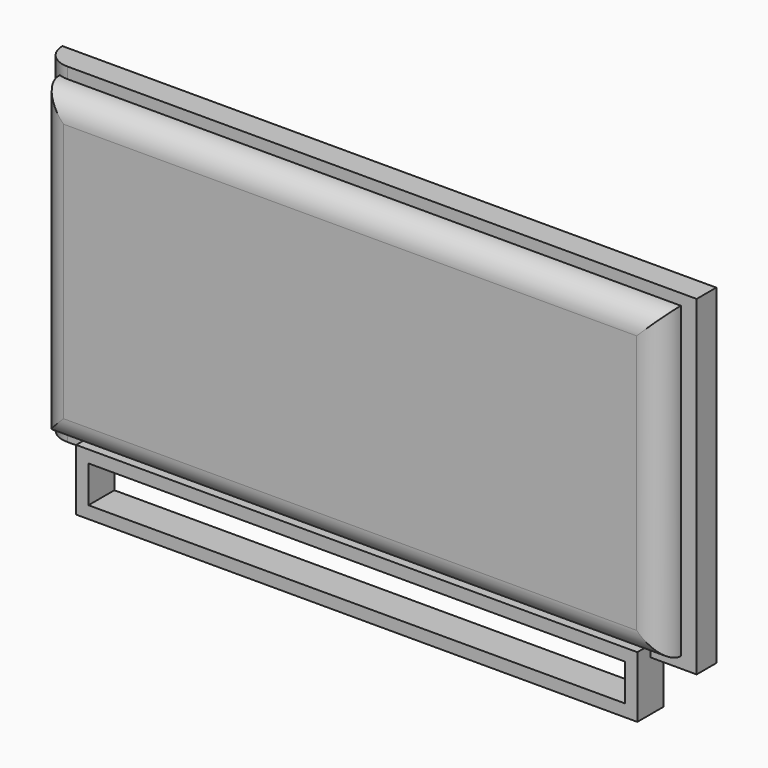
from build123d import *

# Parameters (mm, degrees)
F0_W          = 128.7825703621
F0_H          = 63.8163611293
F1_DEPTH      = 5.08
F0_W_2        = 135.2983415127
F0_H_2        = 68.4157386422
F2_DEPTH      = 5.08
F3_W          = 116.1342710257
F3_H          = 6.7074256949
F4_DEPTH      = 12.7
F5_T          = -2.54
F6_T1_DEPTH   = 89.2163611293
F6_T3_DEPTH   = 154.1825703621
F6_2_T1_DEPTH = 93.8157386422
F7_DEPTH      = 2.54


# Not quite as in the source:
# - a fillet or chamfer that OpenCascade refuses, or shapes differently, is made with other operations: its cross-section is extruded or revolved along the edge and cut away or added


with BuildPart() as f1:
    # F0 (on Front) → F1 (new body)
    with BuildSketch(Plane.XZ):
        Rectangle(F0_W, F0_H)
    extrude(amount=F1_DEPTH)

    # F6: fillet of radius 5.08 on 4 edges, made by hand

    # F6_s2 → F6_t1 (cut)
    with BuildSketch(Plane.XY.offset(-44.6081805646)):
        with BuildLine():
            ThreePointArc((64.391285181, 0), (62.9033876295, -3.5921024484), (59.311285181, -5.08))
            Line((59.311285181, -5.08), (64.391285181, -5.08))
            Line((64.391285181, -5.08), (64.391285181, 0))
        make_face()
        with BuildLine():
            ThreePointArc((-64.391285181, 0), (-62.9033876295, -3.5921024484), (-59.311285181, -5.08))
            Line((-59.311285181, -5.08), (-64.391285181, -5.08))
            Line((-64.391285181, -5.08), (-64.391285181, 0))
        make_face()
    extrude(amount=F6_T1_DEPTH, mode=Mode.SUBTRACT)

    # F6_s4 → F6_t3 (cut)
    with BuildSketch(Plane.YZ.offset(-77.091285181)):
        with BuildLine():
            ThreePointArc((0, 31.9081805646), (-3.5921024484, 30.4202830131), (-5.08, 26.8281805646))
            Line((-5.08, 26.8281805646), (-5.08, 31.9081805646))
            Line((-5.08, 31.9081805646), (0, 31.9081805646))
        make_face()
        with BuildLine():
            ThreePointArc((0, -31.9081805646), (-3.5921024484, -30.4202830131), (-5.08, -26.8281805646))
            Line((-5.08, -26.8281805646), (-5.08, -31.9081805646))
            Line((-5.08, -31.9081805646), (0, -31.9081805646))
        make_face()
    extrude(amount=F6_T3_DEPTH, mode=Mode.SUBTRACT)


with BuildPart() as f2:
    # F0 (on Front) → F2 (new body)
    with BuildSketch(Plane.XZ):
        Rectangle(F0_W_2, F0_H_2)
        Rectangle(F0_W, F0_H, mode=Mode.SUBTRACT)
    extrude(amount=-F2_DEPTH)

    # F6#2: fillet of radius 5.08 on 1 edges, made by hand

    # F6_2_s2 → F6_2_t1 (cut)
    with BuildSketch(Plane.XY.offset(-46.9078693211)):
        with BuildLine():
            ThreePointArc((-67.6491707563, 5.08), (-66.1612732048, 1.4878975516), (-62.5691707563, 0))
            Line((-62.5691707563, 0), (-67.6491707563, 0))
            Line((-67.6491707563, 0), (-67.6491707563, 5.08))
        make_face()
    extrude(amount=F6_2_T1_DEPTH, mode=Mode.SUBTRACT)


with BuildPart() as f4:
    # F3 (on face) → F4 (new body)
    with BuildSketch(Plane(origin=(0, 0, -31.9081805646), x_dir=(1, 0, 0), z_dir=(0, 0, -1))):
        Rectangle(F3_W, F3_H)
    extrude(amount=F4_DEPTH)

    # F5
    f5_openings = [f4.faces().sort_by_distance(p)[0] for p in [
        (0, 3.353713, -38.258181),
        (0, -3.353713, -38.258181),
    ]]
    offset(amount=F5_T, openings=f5_openings)


with BuildPart() as f7:
    # F7 (new): a face of the model
    f7_faces = [f1.part.faces().sort_by_distance(p)[0] for p in [
        (0, 0, 0),
    ]]
    extrude(f7_faces, amount=F7_DEPTH)


solid = Compound([f1.part, f2.part, f4.part, f7.part])
